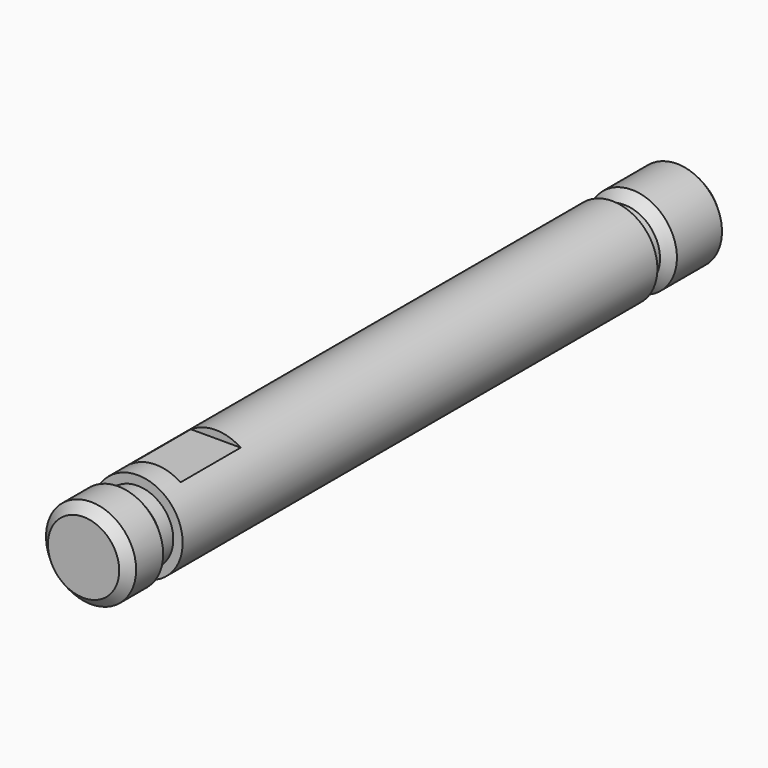
from build123d import *

# Parameters (mm, degrees)
F0_R      = 6
F1_DEPTH  = 7
F2_R      = 4.75
F3_DEPTH  = 2
F4_R      = 6
F5_DEPTH  = 79
F6_R      = 4.75
F7_DEPTH  = 2
F8_R      = 6
F9_DEPTH  = 10
F10_SIZE  = 1.24999
F12_W     = 13
F12_H     = 10
F13_DEPTH = 1


# Not quite as in the source:
# - a fillet or chamfer is up to 0.001 mm smaller than in the source, because OpenCascade refuses the exact size


with BuildPart() as f1:
    # F0 (on Front) → F1 (new body)
    with BuildSketch(Plane.XZ):
        Circle(F0_R)
    extrude(amount=-F1_DEPTH)

    # F2 (on face) → F3 (join)
    with BuildSketch(Plane(origin=(0, 7, 0), x_dir=(-1, 0, 0), z_dir=(0, 1, 0))):
        Circle(F2_R)
    extrude(amount=F3_DEPTH)

    # F4 (on face) → F5 (join)
    with BuildSketch(Plane(origin=(0, 9, 0), x_dir=(-1, 0, 0), z_dir=(0, 1, 0))):
        Circle(F4_R)
    extrude(amount=F5_DEPTH)

    # F6 (on face) → F7 (join)
    with BuildSketch(Plane(origin=(0, 88, 0), x_dir=(-1, 0, 0), z_dir=(0, 1, 0))):
        Circle(F6_R)
    extrude(amount=F7_DEPTH)

    # F8 (on face) → F9 (join)
    with BuildSketch(Plane(origin=(0, 90, 0), x_dir=(-1, 0, 0), z_dir=(0, 1, 0))):
        Circle(F8_R)
    extrude(amount=F9_DEPTH)

    # F10 (size 1.25 in the source; OpenCascade refuses exactly that, so slightly less here)
    f10_edges = [f1.edges().sort_by_distance(p)[0] for p in [
        (6, 3.5, 0),
        (-6, 0, 0),
        (-6, 7, 0),
        (-6, 95, 0),
        (6, 90, 0),
        (6, 100, 0),
    ]]
    chamfer(f10_edges, length=F10_SIZE)

    # F12 (on offset) → F13 (cut)
    with BuildSketch(Plane.XY.offset(6)):
        with Locations((0, 17)):
            Rectangle(F12_W, F12_H)
    f13 = extrude(amount=-F13_DEPTH, mode=Mode.SUBTRACT)

    # F14: F13 across plane
    add(f13.mirror(Plane.XY), mode=Mode.SUBTRACT)


solid = f1.part
